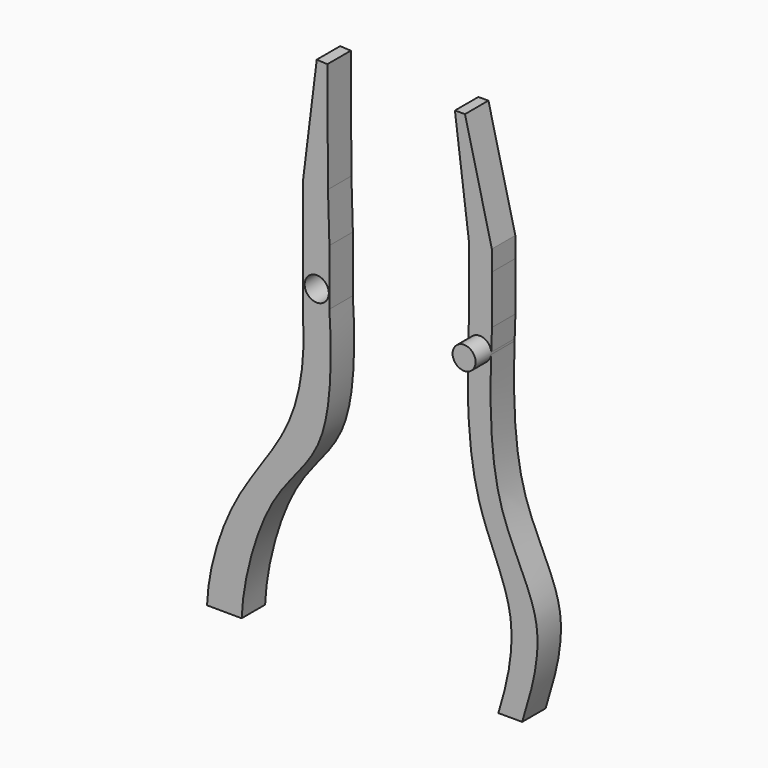
from build123d import *

# Parameters (mm, degrees)
F1_DEPTH = 7.62
F2_DEPTH = 7.62
F3_R     = 2.9931989814
F5_DEPTH = 12.7
F3_R_2   = 3.7293138993
F6_DEPTH = 25.4
F8_DEPTH = 25.4


# Not quite as in the source:
# - the program builds the solid bodies; features that only make, move or delete a surface that nothing else refers to are left out


with BuildPart() as f1:
    # F0 (on Front) → F1 (new body)
    with BuildSketch(Plane.XZ):
        with BuildLine():
            add(Edge.make_bspline(
                [(39.446875453, -16.3293741643), (41.9001167123, -8.2704796171), (45.5947084864, 8.0337070769), (33.0409793146, 28.1137801453), (31.5653655238, 47.3073931738), (31.5021629172, 56.4661241863)],
                knots=[0, 0, 0, 0, 0.3011805087, 0.61146441, 0.8692310246, 0.8692310246, 0.8692310246, 0.8692310246], degree=3))
            Line((39.446875453, -16.3293741643), (45.644475453, -16.3293741643))
            add(Edge.make_bspline(
                [(45.644475453, -16.3293741643), (48.0836032329, -8.303541327), (53.0592723839, 8.1631929353), (36.5013753886, 30.9253527959), (37.2587382897, 57.1631543308), (37.7889908314, 71.3900855683)],
                knots=[0, 0, 0, 0, 0.2999480229, 0.6102007791, 1, 1, 1, 1], degree=3))
            Line((37.7889908314, 71.3900855683), (37.7889908314, 84.0900855683))
            Line((37.7889908314, 84.0900855683), (37.7582089288, 89.353502548))
            Line((37.7582089288, 89.353502548), (30.7703027195, 117.9347286346))
            Line((30.7703027195, 117.9347286346), (28.1520184027, 117.9194161915))
            Line((28.1520184027, 117.9194161915), (31.7724533379, 89.3184962116))
            Line((31.7724533379, 89.3184962116), (31.7724533379, 83.3474483013))
            Line((31.7724533379, 83.3474483013), (31.7724533379, 70.6474483013))
            add(Edge.make_bspline(
                [(31.5021629172, 56.4661241863), (31.470099261, 61.1124895525), (31.5941022469, 65.8744563999), (31.7724533379, 70.6474483013)],
                knots=[0.8692310246, 0.8692310246, 0.8692310246, 0.8692310246, 1, 1, 1, 1], degree=3))
        make_face()
    extrude(amount=F1_DEPTH)

    # F3 (on Front) → F5 (join)
    with BuildSketch(Plane.XZ):
        with Locations((34.6025004983, 65.4727444053)):
            Circle(F3_R)
    extrude(amount=F5_DEPTH)

    # F3 (on Front) → F6 (cut)
    with BuildSketch(Plane.XZ):
        with Locations((-7.5630368665, 65.4727444053)):
            Circle(F3_R_2)
    extrude(amount=-F6_DEPTH, mode=Mode.SUBTRACT)


with BuildPart() as f2:
    # F0 (on Front) → F2 (new body)
    with BuildSketch(Plane.XZ):
        with BuildLine():
            add(Edge.make_bspline(
                [(-36.291336976, -16.2931783742), (-35.9797269437, -7.4434377304), (-30.0480350171, 12.015348302), (-13.0050265683, 30.9384280949), (-10.7868187806, 48.4065419002), (-11.3293034956, 57.1104250848)],
                knots=[0, 0, 0, 0, 0.3461239889, 0.6727746853, 1, 1, 1, 1], degree=3))
            Line((-36.291336976, -16.2931783742), (-27.2889714688, -16.3293741643))
            add(Edge.make_bspline(
                [(-27.2889714688, -16.3293741643), (-26.9699991675, -7.2705447074), (-20.9702017655, 15.7077591395), (-3.4595302989, 28.7919953348), (-3.9001260053, 52.4256435308), (-4.4848158276, 61.8066855623)],
                knots=[0, 0, 0, 0, 0.3543017036, 0.6473166786, 1, 1, 1, 1], degree=3))
            Line((-4.4848158276, 61.8066855623), (-4.4748519132, 76.4043473555))
            Line((-4.4748519132, 76.4043473555), (-4.8449948946, 89.1043473555))
            Line((-4.8449948946, 89.1043473555), (-5.0123790024, 117.7254617214))
            Line((-5.0123790024, 117.7254617214), (-7.7673349517, 117.8813783243))
            Line((-7.7673349517, 117.8813783243), (-11.3293034956, 89.1043473555))
            Line((-11.3293034956, 89.1043473555), (-11.3293034956, 85.981985124))
            Line((-11.3293034956, 85.981985124), (-11.3293034956, 79.6000332555))
            Line((-11.3293034956, 79.6000332555), (-11.3221835393, 70.6508324852))
            Line((-11.3221835393, 70.6508324852), (-11.3293034956, 57.1104250848))
        make_face()
    extrude(amount=F2_DEPTH)

    # F7 (on face) → F8 (cut)
    with BuildSketch(Plane.XZ.offset(7.62)):
        with BuildLine():
            ThreePointArc((-7.6848294678, 68.5448205068), (-10.0162462779, 63.2158830381), (-4.627879267, 65.4064491391))
            ThreePointArc((-4.627879267, 65.4064491391), (-5.5184236255, 67.5970152401), (-7.6848294678, 68.5448205068))
        make_face()
    extrude(amount=-F8_DEPTH, mode=Mode.SUBTRACT)


solid = Compound([f1.part, f2.part])
